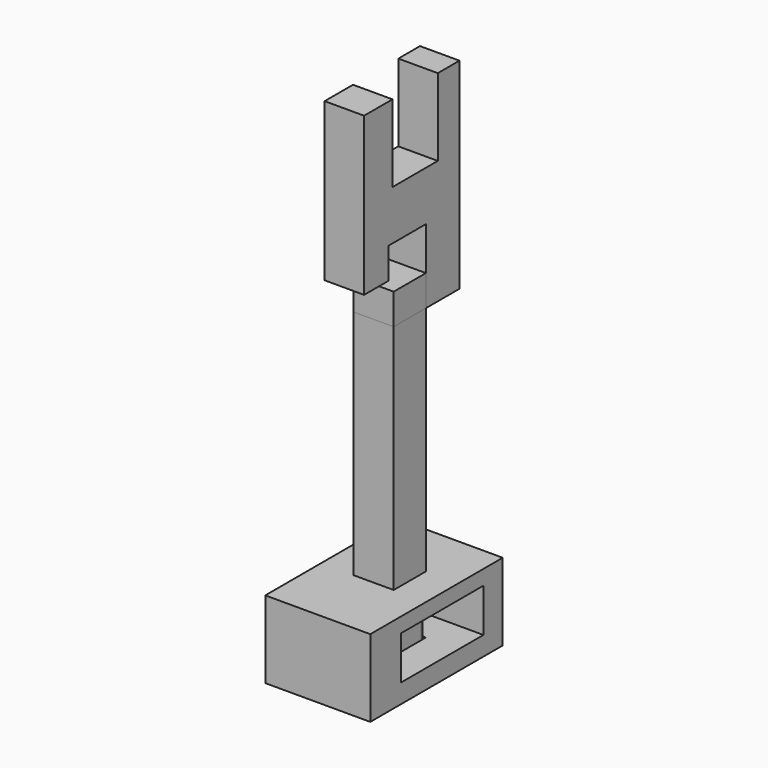
from build123d import *

# Parameters (mm, degrees)
F0_W      = 13.0280144513
F0_H      = 13.0280144513
F1_DEPTH  = 75
F2_W      = 33.9875258505
F2_H      = 53.5712684505
F2_W_2    = 13.0280144513
F2_H_2    = 13.0280144513
F3_DEPTH  = 25
F4_DEPTH  = 25
F5_W      = 33.3761908114
F5_H      = 14.0360295773
F6_DEPTH  = 34
F7_W      = 12.7713497204
F7_H      = 13.5793518275
F8_DEPTH  = 25
F9_DEPTH  = 10
F10_DEPTH = 15
F11_W     = 12.7713497204
F11_H     = 16.0501429439
F12_DEPTH = 25
F13_W     = 12.7713497204
F13_H     = 9.8180785775
F14_DEPTH = 10
F15_W     = 12.7713497204
F15_H     = 11.4813564345
F16_DEPTH = 25
F17_W     = 12.7713497204
F17_H     = 8.7616005912
F18_DEPTH = 25
F19_R     = 2
F20_R     = 2


with BuildPart() as f1:
    # F0 (on Top) → F1 (new body)
    with BuildSketch(Plane.XY):
        Rectangle(F0_W, F0_H)
    extrude(amount=F1_DEPTH)


with BuildPart() as f3:
    # F2 (on face) → F3 (new body)
    with BuildSketch(Plane(origin=(0, 0, 0), x_dir=(1, 0, 0), z_dir=(0, 0, -1))):
        with Locations((0, 2.289036056)):
            Rectangle(F2_W, F2_H)
        Rectangle(F2_W_2, F2_H_2, mode=Mode.SUBTRACT)
    extrude(amount=F3_DEPTH)

    # F5 (on face) → F6 (cut)
    with BuildSketch(Plane.YZ.offset(16.9937629253)):
        with Locations((0, -11.8051227182)):
            Rectangle(F5_W, F5_H)
    extrude(amount=-F6_DEPTH, mode=Mode.SUBTRACT)


with BuildPart() as f4:
    # F4 (new): a face of the model
    f4_faces = [f1.part.faces().sort_by_distance(p)[0] for p in [
        (0, 0, 0),
    ]]
    extrude(f4_faces, amount=F4_DEPTH)

    # F19
    f19_edges = [f4.edges().sort_by_distance(p)[0] for p in [
        (6.514007, -6.514007, -12.5),
        (6.514007, 6.514007, -12.5),
        (6.514007, 0, 0),
        (6.514007, 0, -25),
    ]]
    fillet(f19_edges, radius=F19_R)

    # F20
    f20_edges = [f4.edges().sort_by_distance(p)[0] for p in [
        (-6.514007, 6.514007, -12.5),
        (-6.514007, -6.514007, -12.5),
        (-6.514007, 0, 0),
        (-6.514007, 0, -25),
    ]]
    fillet(f20_edges, radius=F20_R)


with BuildPart() as f8:
    # F7 (on face) → F8 (new body)
    with BuildSketch(Plane.XY.offset(75)):
        with Locations((0.1283323654, 13.3036831394)):
            Rectangle(F7_W, F7_H)
    extrude(amount=F8_DEPTH)

    # F10 (add): a face of the model
    f10_faces = [f8.faces().sort_by_distance(p)[0] for p in [
        (0.1283323654, 13.3036831394, 100),
    ]]
    extrude(f10_faces, amount=F10_DEPTH)

    # F11 (on face) → F12 (join)
    with BuildSketch(Plane.XZ.offset(-6.5140072256)):
        with Locations((0.1283323654, 106.9749285281)):
            Rectangle(F11_W, F11_H)
    extrude(amount=F12_DEPTH)

    # F13 (on face) → F14 (join)
    with BuildSketch(Plane(origin=(0, 0, 98.9498570561), x_dir=(1, 0, 0), z_dir=(0, 0, -1))):
        with Locations((0.1283323654, 13.5769534856)):
            Rectangle(F13_W, F13_H)
    extrude(amount=F14_DEPTH)

    # F15 (on face) → F16 (join)
    with BuildSketch(Plane.XY.offset(115)):
        with Locations((0.1283323654, -12.7453145571)):
            Rectangle(F15_W, F15_H)
    extrude(amount=F16_DEPTH)

    # F17 (on face) → F18 (join)
    with BuildSketch(Plane.XY.offset(115)):
        with Locations((0.1283323654, 15.7125587575)):
            Rectangle(F17_W, F17_H)
    extrude(amount=F18_DEPTH)


with BuildPart() as f9:
    # F9 (new): a face of the model
    f9_faces = [f1.part.faces().sort_by_distance(p)[0] for p in [
        (0, 0, 75),
    ]]
    extrude(f9_faces, amount=F9_DEPTH)


solid = Compound([f1.part, f3.part, f4.part, f8.part, f9.part])
